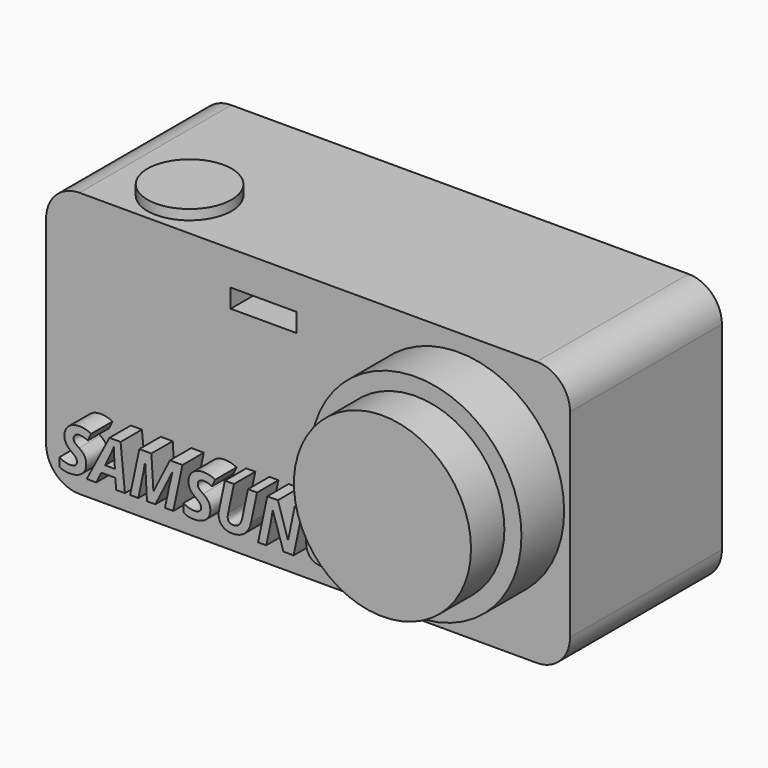
from build123d import *

# Parameters (mm, degrees)
F0_W         = 79.8008386046
F0_H         = 28.9090070873
F1_DEPTH     = 40.386
F2_R         = 16.0900860403
F3_DEPTH     = 8.128
F4_R         = 5.08
F5_R         = 13.4881290769
F6_DEPTH     = 6.35
F7_R         = 9.7378427485
F8_DEPTH     = 25.4
F9_TEXT_SIZE = 9.2742192693
F10_DEPTH    = 4.064
F11_W        = 10.0486502051
F11_H        = 2.8439573944
F12_DEPTH    = 28.702
F13_R        = 6.4057502918
F14_DEPTH    = 1.524


# Not quite as in the source:
# - Text() gives the source's letters only with a copy of the font that has no kerning and outlines rounded to 1/6400 em; it was checked with that copy


with BuildPart() as f1:
    # F0 (on Top) → F1 (new body)
    with BuildSketch(Plane.XY):
        with Locations((19.8422102258, 14.4545035437)):
            Rectangle(F0_W, F0_H)
    extrude(amount=F1_DEPTH)

    # F2 (on face) → F3 (join)
    with BuildSketch(Plane.XZ):
        with Locations((42.7541583776, 21.7088758945)):
            Circle(F2_R)
    extrude(amount=F3_DEPTH)

    # F4
    f4_edges = [f1.edges().sort_by_distance(p)[0] for p in [
        (-20.058209, 14.454504, 40.386),
        (-20.058209, 14.454504, 0),
        (59.74263, 14.454504, 40.386),
        (59.74263, 14.454504, 0),
    ]]
    fillet(f4_edges, radius=F4_R)

    # F5 (on face) → F6 (join)
    with BuildSketch(Plane.XZ.offset(8.128)):
        with Locations((42.7541583776, 21.7088758945)):
            Circle(F5_R)
    extrude(amount=F6_DEPTH)

    # F7 (on face) → F8 (join)
    with BuildSketch(Plane.XZ.offset(14.478)):
        with Locations((42.7541583776, 21.7088758945)):
            Circle(F7_R)
    extrude(amount=-F8_DEPTH)

    # F9 (on face) → F10 (join)
    with BuildSketch(Plane.XZ):
        with Locations((-14.9782090765, 5.08)):
            Text('SAMSUNG', F9_TEXT_SIZE, font='Open Sans', font_style=FontStyle.BOLDITALIC, text_align=(TextAlign.LEFT, TextAlign.BOTTOM))
    extrude(amount=F10_DEPTH)

    # F11 (on face) → F12 (cut)
    with BuildSketch(Plane.XZ):
        with Locations((13.0822043866, 33.7482932955)):
            Rectangle(F11_W, F11_H)
    extrude(amount=-F12_DEPTH, mode=Mode.SUBTRACT)

    # F13 (on face) → F14 (join)
    with BuildSketch(Plane.XY.offset(40.386)):
        with Locations((-4.3040299788, 7.6210005209)):
            Circle(F13_R)
    extrude(amount=F14_DEPTH)


solid = f1.part
